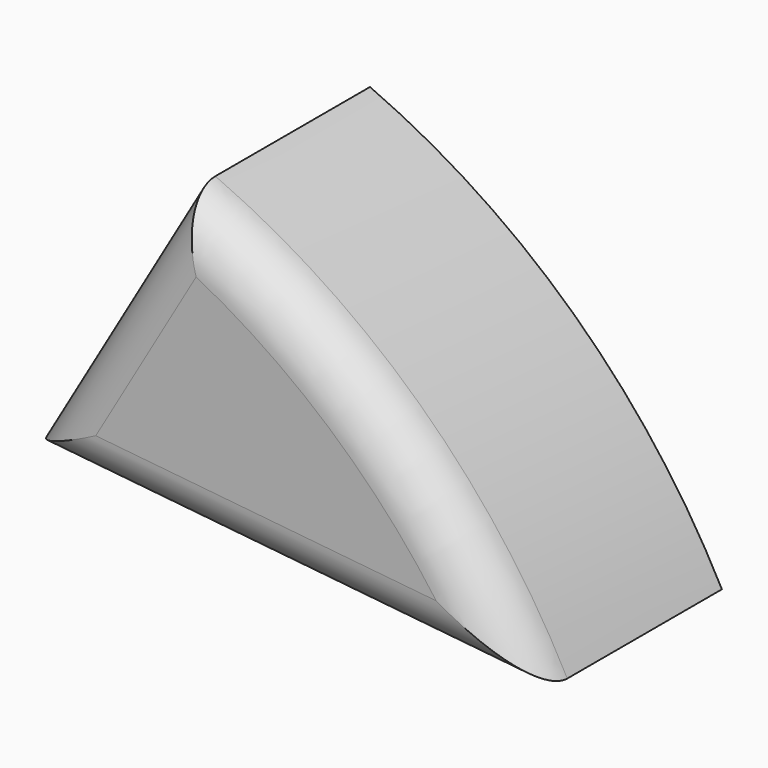
from build123d import *

# Parameters (mm, degrees)
F1_DEPTH    = 25.4
F2_T1_DEPTH = 355.0052962601
F3_T1_DEPTH = 79.5444841249
F3_T3_DEPTH = 58.9324911013
F3_T6_ANGLE = 57.8558117321


# Not quite as in the source:
# - a fillet or chamfer that OpenCascade refuses, or shapes differently, is made with other operations: its cross-section is extruded or revolved along the edge and cut away or added


with BuildPart() as f1:
    # F0 (on Front) → F1 (new body)
    with BuildSketch(Plane.XZ):
        Polygon((16.8645065278, 28.9830360562), (0, 0), (62.5720471144, -6.3669001684), (62.5720471144, 25.0710807741), align=None)
    extrude(amount=F1_DEPTH)

    # F2: fillet of radius 76.2 on 1 edges, made by hand

    # F2_s2 → F2_t1 (cut)
    with BuildSketch(Plane.XZ.offset(-164.8026481301)):
        with BuildLine():
            ThreePointArc((62.5720471144, -40.849978478), (50.1292639894, 0.8807930983), (16.8645065278, 28.9830360562))
            Line((16.8645065278, 28.9830360562), (62.5720471144, 25.0710807741))
            Line((62.5720471144, 25.0710807741), (62.5720471144, -40.849978478))
        make_face()
    extrude(amount=F2_T1_DEPTH, mode=Mode.SUBTRACT)

    # F3: fillet of radius 5.08 on 3 edges, made by hand

    # F3_s2 → F3_t1 (cut)
    with BuildSketch(Plane(origin=(-12.6347602087, 0, 1.2856261), x_dir=(0, 1, 0), z_dir=(0.9948630086, 0, -0.1012304016))):
        with BuildLine():
            ThreePointArc((-20.32, 0), (-23.9121024484, 1.4878975516), (-25.4, 5.08))
            Line((-25.4, 5.08), (-25.4, 0))
            Line((-25.4, 0), (-20.32, 0))
        make_face()
    extrude(amount=F3_T1_DEPTH, mode=Mode.SUBTRACT)

    # F3_s4 → F3_t3 (cut)
    with BuildSketch(Plane(origin=(23.2517216099, 0, 39.9599884335), x_dir=(0, 1, 0), z_dir=(-0.5029303214, 0, -0.8643269588))):
        with BuildLine():
            ThreePointArc((-20.32, 0), (-23.9121024484, 1.4878975516), (-25.4, 5.08))
            Line((-25.4, 5.08), (-25.4, 0))
            Line((-25.4, 0), (-20.32, 0))
        make_face()
    extrude(amount=F3_T3_DEPTH, mode=Mode.SUBTRACT)

    # F3_s5 → F3_t6 (revolve, cut)
    with BuildSketch(Plane(origin=(-3.2129562092, 0, 0.8033671188), x_dir=(0, 1, 0), z_dir=(-0.9701334009, 0, 0.2425720192))):
        with BuildLine():
            ThreePointArc((-20.32, -33.2643114045), (-23.9121024484, -31.776413853), (-25.4, -28.1843114045))
            Line((-25.4, -28.1843114045), (-25.4, -33.2643114045))
            Line((-25.4, -33.2643114045), (-20.32, -33.2643114045))
        make_face()
    revolve(axis=Axis((-13.6279528859, -25.4, -40.8499784781), (0, 1, 0)), revolution_arc=F3_T6_ANGLE, mode=Mode.SUBTRACT)


solid = f1.part
